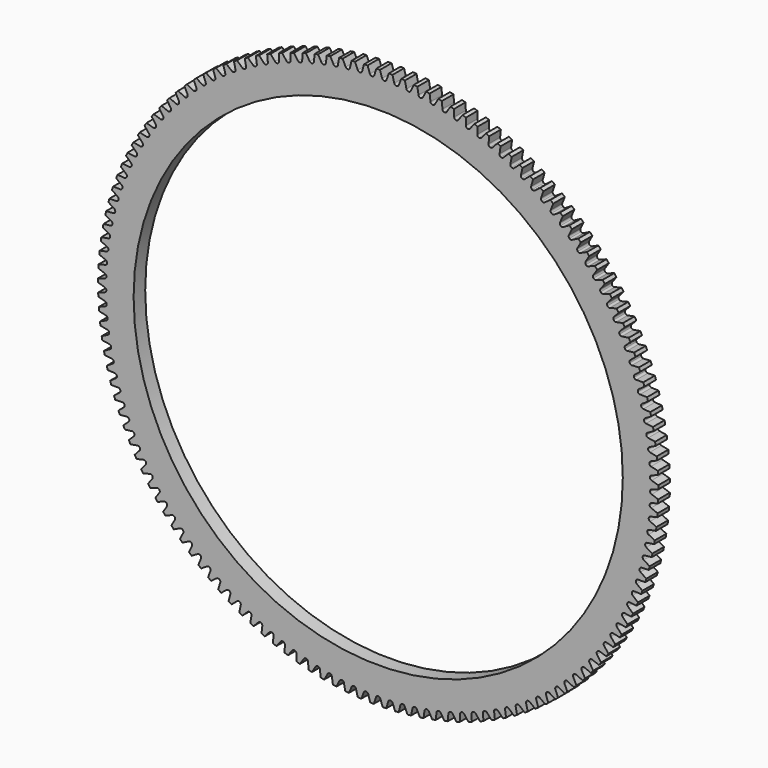
from build123d import *

# Parameters (mm, degrees)
F0_R     = 135
F1_DEPTH = 8


# Not quite as in the source:
# - ends of sketch curves that miss each other by under 0.0002 mm in the source are joined


with BuildPart() as f1:
    # F0 (on Front) → F1 (new body)
    with BuildSketch(Plane.XZ):
        with BuildLine():
            Line((2.149657, 150.904207), (1.001008, 154.59676))
            ThreePointArc((1.001008, 154.59676), (0, 154.6), (-1.0010079954, 154.5967592901))
            Line((-1.0010079954, 154.5967592901), (-2.149657, 150.904207))
            ThreePointArc((-2.149657, 150.904207), (-2.6021653574, 150.2688665421), (-3.343241, 150.025498))
            ThreePointArc((-3.343241, 150.025498), (-4.0944228128, 150.2356123099), (-4.5747845974, 150.8501647845))
            Line((-4.5747845974, 150.8501647845), (-5.886784, 154.487883))
            ThreePointArc((-5.886784, 154.487883), (-6.886942844, 154.4465280227), (-7.8868129881, 154.3986987668))
            Line((-7.8868129881, 154.3986987668), (-8.86983, 150.658644))
            ThreePointArc((-8.86983, 150.658644), (-9.2935865986, 150.003775549), (-10.0230859935, 149.7276358548))
            ThreePointArc((-10.0230859935, 149.7276358548), (-10.7828816043, 149.9040794817), (-11.2901424606, 150.4966232222))
            Line((-11.2901424606, 150.4966232222), (-12.762889, 154.072284))
            ThreePointArc((-12.762889, 154.072284), (-13.7602129304, 153.986416739), (-14.7569599887, 153.8940938824))
            Line((-14.7569599887, 153.8940938824), (-15.572393, 150.113961))
            ThreePointArc((-15.572393, 150.113961), (-15.9665572146, 149.4408662135), (-16.6830310003, 149.1325040036))
            ThreePointArc((-16.6830310003, 149.1325040036), (-17.4499321725, 149.2749258512), (-17.9830853746, 149.8442842908))
            Line((-17.9830853746, 149.8442842908), (-19.613655, 153.350789))
            ThreePointArc((-19.613655, 153.350789), (-20.6061634232, 153.2205796523), (-21.597807937, 153.0839465532))
            Line((-21.597807937, 153.0839465532), (-22.244039, 149.271242))
            ThreePointArc((-22.244039, 149.271242), (-22.6078267089, 148.5812559997), (-23.3098530061, 148.2412830456))
            ThreePointArc((-23.3098530061, 148.2412830456), (-24.0823376284, 148.3493999375), (-24.6403250099, 148.8944429949))
            Line((-24.6403250099, 148.8944429949), (-26.425479, 152.324831))
            ThreePointArc((-26.425479, 152.324831), (-27.4112015967, 152.1505373866), (-28.3957750559, 151.9698652989))
            Line((-28.3957750559, 151.9698652989), (-28.871521, 148.132158))
            ThreePointArc((-28.871521, 148.132158), (-29.2042107107, 147.4266515424), (-29.8903949713, 147.0557428405))
            ThreePointArc((-29.8903949713, 147.0557428405), (-30.6669292534, 147.1293407731), (-31.248642951, 147.6489860283))
            Line((-31.248642951, 147.6489860283), (-33.184838, 150.996446))
            ThreePointArc((-33.184838, 150.996446), (-34.1618180079, 150.7784142057), (-35.1373659455, 150.5540617666))
            Line((-35.1373659455, 150.5540617666), (-35.441681, 146.698971))
            ThreePointArc((-35.441681, 146.698971), (-35.7426132223, 145.9793450273), (-36.411593028, 145.5782371237))
            ThreePointArc((-36.411593028, 145.5782371237), (-37.1906350912, 145.6171701649), (-37.7949198522, 146.1103860945))
            Line((-37.7949198522, 146.1103860945), (-39.878311, 149.368271))
            ThreePointArc((-39.878311, 149.368271), (-40.8446086877, 149.1069345844), (-41.8091940714, 148.8393472543))
            Line((-41.8091940714, 148.8393472543), (-41.941475, 144.974527))
            ThreePointArc((-41.941475, 144.974527), (-42.2100519967, 144.2422097491), (-42.8605001177, 143.8116994298))
            ThreePointArc((-42.8605001177, 143.8116994298), (-43.6405023802, 143.8158899986), (-44.2661578786, 144.2816970855))
            Line((-44.2661578786, 144.2816970855), (-46.49261, 147.443539))
            ThreePointArc((-46.49261, 147.443539), (-47.4463065751, 147.1394168548), (-48.3980139989, 146.8291259967))
            Line((-48.3980139989, 146.8291259967), (-48.357999, 142.96225))
            ThreePointArc((-48.357999, 142.96225), (-48.5936858817, 142.218695529), (-49.2243099488, 141.7596368411))
            ThreePointArc((-49.2243099488, 141.7596368411), (-50.0037248855, 141.7290762238), (-50.649509867, 142.1665501028))
            Line((-50.649509867, 142.1665501028), (-53.014602, 145.226072))
            ThreePointArc((-53.014602, 145.226072), (-53.9538044342, 144.8797673489), (-54.8907449336, 144.5273888252))
            Line((-54.8907449336, 144.5273888252), (-54.678511, 140.666134))
            ThreePointArc((-54.678511, 140.666134), (-54.8808417827, 139.9128185145), (-55.4903900412, 139.4261231106))
            ThreePointArc((-55.4903900412, 139.4261231106), (-56.267670189, 139.3608729051), (-56.9323022426, 139.7691447946))
            Line((-56.9323022426, 139.7691447946), (-59.431339, 142.720272))
            ThreePointArc((-59.431339, 142.720272), (-60.3541820807, 142.3324724206), (-61.274495002, 141.9387060046))
            Line((-61.274495002, 141.9387060046), (-60.890465, 138.090739))
            ThreePointArc((-60.890465, 138.090739), (-61.0590363601, 137.3291573655), (-61.6462997807, 136.8157914828))
            ThreePointArc((-61.6462997807, 136.8157914828), (-62.4199014329, 136.7159810346), (-63.1020606883, 137.0942402888))
            Line((-63.1020606883, 137.0942402888), (-65.73008, 139.931114))
            ThreePointArc((-65.73008, 139.931114), (-66.6347317571, 139.5025896665), (-67.5365900447, 139.068217092))
            Line((-67.5365900447, 139.068217092), (-66.981527, 135.241177))
            ThreePointArc((-66.981527, 135.241177), (-67.116004748, 134.4728427274), (-67.6798160822, 133.9338261721))
            ThreePointArc((-67.6798160822, 133.9338261721), (-68.448203257, 133.7996526891), (-69.1465355867, 134.1471484186))
            Line((-69.1465355867, 134.1471484186), (-71.89832, 136.864136))
            ThreePointArc((-71.89832, 136.864136), (-72.7829839253, 136.3957376568), (-73.6645967253, 135.9216214931))
            Line((-73.6645967253, 135.9216214931), (-72.939602, 132.123106))
            ThreePointArc((-72.939602, 132.123106), (-73.039719853, 131.3495439601), (-73.5789597097, 130.7859464559))
            ThreePointArc((-73.5789597097, 130.7859464559), (-74.3406074994, 130.617677222), (-75.0537266479, 130.9337193899))
            Line((-75.0537266479, 130.9337193899), (-77.923812, 133.525427))
            ThreePointArc((-77.923812, 133.525427), (-78.7867323418, 133.0180845107), (-79.6463498584, 132.5051657644))
            Line((-79.6463498584, 132.5051657644), (-78.752863, 128.742718))
            ThreePointArc((-78.752863, 128.742718), (-78.8184219814, 127.9654637065), (-79.3320200625, 127.3784041055))
            ThreePointArc((-79.3320200625, 127.3784041055), (-80.0854159326, 127.1763722155), (-80.8119061154, 127.4603338601))
            Line((-80.8119061154, 127.4603338601), (-83.794594, 129.921615))
            ThreePointArc((-83.794594, 129.921615), (-84.6340575656, 129.3763359351), (-85.4699729956, 128.8256329933))
            Line((-85.4699729956, 128.8256329933), (-84.409768, 125.106722))
            ThreePointArc((-84.409768, 125.106722), (-84.4406376429, 124.3273190288), (-84.9275740807, 123.7179631234))
            ThreePointArc((-84.9275740807, 123.7179631234), (-85.6712217244, 123.4825711451), (-86.4096396772, 123.7338874287))
            Line((-86.4096396772, 123.7338874287), (-89.49901, 126.059856))
            ThreePointArc((-89.49901, 126.059856), (-90.3133495837, 125.4777226721), (-91.1239030464, 124.8903290635))
            Line((-91.1239030464, 124.8903290635), (-89.899085, 121.222339))
            ThreePointArc((-89.899085, 121.222339), (-89.8952036419, 120.4423345066), (-90.3545119051, 119.8118918681))
            ThreePointArc((-90.3545119051, 119.8118918681), (-91.0869354192, 119.5436056884), (-91.8358161037, 119.7617788486))
            Line((-91.8358161037, 119.7617788486), (-95.025734, 121.947817))
            ThreePointArc((-95.025734, 121.947817), (-95.8133327272, 121.3299850478), (-96.5969149772, 120.7070669716))
            Line((-96.5969149772, 120.7070669716), (-95.209915, 117.09728))
            ThreePointArc((-95.209915, 117.09728), (-95.1712903771, 116.3182224536), (-95.6020587486, 115.6679446817))
            ThreePointArc((-95.6020587486, 115.6679446817), (-96.3218043226, 115.3672985935), (-97.079660293, 115.5518945287))
            Line((-97.079660293, 115.5518945287), (-100.363793, 117.593661))
            ThreePointArc((-100.363793, 117.593661), (-101.1230871147, 116.9413581775), (-101.87814188, 116.284152863))
            Line((-101.87814188, 116.284152863), (-100.331715, 112.739735))
            ThreePointArc((-100.331715, 112.739735), (-100.2584245046, 111.9631717029), (-100.6597973494, 111.2943504041))
            ThreePointArc((-100.6597973494, 111.2943504041), (-101.3654352267, 110.9619395838), (-102.1307622583, 111.11259254))
            Line((-102.1307622583, 111.11259254), (-105.502588, 113.006035))
            ThreePointArc((-105.502588, 113.006035), (-106.2320709678, 112.3205550996), (-106.9571003273, 111.6303663416))
            Line((-106.9571003273, 111.6303663416), (-105.254315, 108.158356))
            ThreePointArc((-105.254315, 108.158356), (-105.1465047957, 107.3858283151), (-105.5176853011, 106.6997913183))
            ThreePointArc((-105.5176853011, 106.6997913183), (-106.2078145762, 106.3362765517), (-106.9790928527, 106.452687292))
            Line((-106.9790928527, 106.452687292), (-110.431919, 108.194045))
            ThreePointArc((-110.431919, 108.194045), (-111.1301414659, 107.4767493822), (-111.8237051815, 106.7549481733))
            Line((-111.8237051815, 106.7549481733), (-109.967943, 103.362238))
            ThreePointArc((-109.967943, 103.362238), (-109.8258253179, 102.5952799651), (-110.16607692, 101.8933889227))
            ThreePointArc((-110.16607692, 101.8933889227), (-110.8393276966, 101.4994917148), (-111.6150261855, 101.5814285874))
            Line((-111.6150261855, 101.5814285874), (-115.141996, 103.167246))
            ThreePointArc((-115.141996, 103.167246), (-115.8075727738, 102.4195591098), (-116.468294186, 101.6675781624))
            Line((-116.468294186, 101.6675781624), (-114.46324, 98.360904))
            ThreePointArc((-114.46324, 98.360904), (-114.2870972871, 97.6010385417), (-114.5957441497, 96.8846871324))
            ThreePointArc((-114.5957441497, 96.8846871324), (-115.2507797841, 96.461189931), (-116.0293581746, 96.5084905603))
            Line((-116.0293581746, 96.5084905603), (-119.623471, 97.935618))
            ThreePointArc((-119.623471, 97.935618), (-120.2550791172, 97.1590240097), (-120.8816459047, 96.378356924))
            Line((-120.8816459047, 96.378356924), (-118.73128, 93.164284))
            ThreePointArc((-118.73128, 93.164284), (-118.5214630535, 92.4130193699), (-118.7978919781, 91.6836299823))
            ThreePointArc((-118.7978919781, 91.6836299823), (-119.4334124107, 91.2313737423), (-120.2133249965, 91.2439440102))
            Line((-120.2133249965, 91.2439440102), (-123.867443, 92.509548))
            ThreePointArc((-123.867443, 92.509548), (-124.463829999, 91.7055888263), (-125.0549987572, 90.8977848235))
            Line((-125.0549987572, 90.8977848235), (-122.763591, 87.782695))
            ThreePointArc((-122.763591, 87.782695), (-122.5205160981, 87.0415226788), (-122.7641784334, 86.3005433193))
            ThreePointArc((-122.7641784334, 86.3005433193), (-123.3789207173, 85.8204254609), (-124.1586188106, 85.7982406375))
            Line((-124.1586188106, 85.7982406375), (-127.865489, 86.899809))
            ThreePointArc((-127.865489, 86.899809), (-128.4254694957, 86.0700806599), (-128.9800661266, 85.2367440837))
            Line((-128.9800661266, 85.2367440837), (-126.552166, 82.226821))
            ThreePointArc((-126.552166, 82.226821), (-126.2763149288, 81.4972130945), (-126.4867268393, 80.7461148923))
            ThreePointArc((-126.4867268393, 80.7461148923), (-127.0794716473, 80.2390882407), (-127.8574081662, 80.1821923334))
            Line((-127.8574081662, 80.1821923334), (-131.609669, 81.117538))
            ThreePointArc((-131.609669, 81.117538), (-132.1321322996, 80.2636880161), (-132.6490559667, 79.4064729801))
            Line((-132.6490559667, 79.4064729801), (-130.089483, 76.507694))
            ThreePointArc((-130.089483, 76.507694), (-129.7814040716, 75.7910982673), (-129.9581484083, 75.031372248))
            ThreePointArc((-129.9581484083, 75.031372248), (-130.5277186577, 74.4984447725), (-131.3023479981, 74.4069510095))
            Line((-131.3023479981, 74.4069510095), (-135.092551, 75.174216))
            ThreePointArc((-135.092551, 75.174216), (-135.5764588793, 74.297939391), (-136.0546831234, 73.4185480666))
            Line((-136.0546831234, 73.4185480666), (-133.368519, 70.636668))
            ThreePointArc((-133.368519, 70.636668), (-133.0288242558, 69.9345070672), (-133.1715496027, 69.1676617823))
            ThreePointArc((-133.1715496027, 69.1676617823), (-133.7168142387, 68.6098905207), (-134.4865989963, 68.4839800237))
            Line((-134.4865989963, 68.4839800237), (-138.307218, 69.081643))
            ThreePointArc((-138.307218, 69.081643), (-138.7516105774, 68.1846798203), (-139.1901860152, 67.2848580073))
            Line((-139.1901860152, 67.2848580073), (-136.382765, 64.625399))
            ThreePointArc((-136.382765, 64.625399), (-136.0121281444, 63.9390677035), (-136.120551355, 63.166625683))
            ThreePointArc((-136.120551355, 63.166625683), (-136.6404271667, 62.5851179456), (-137.4038389928, 62.4250410646))
            Line((-137.4038389928, 62.4250410646), (-141.24729, 62.851914))
            ThreePointArc((-141.24729, 62.851914), (-141.6512843299, 61.936044818), (-142.049340174, 61.0175790747))
            Line((-142.049340174, 61.0175790747), (-139.126235, 58.485822))
            ThreePointArc((-139.126235, 58.485822), (-138.7253925624, 57.8166829615), (-138.7992984203, 57.0401781838))
            ThreePointArc((-138.7992984203, 57.0401781838), (-139.2927539466, 56.4360890513), (-140.0482769559, 56.2421636668))
            Line((-140.0482769559, 56.2421636668), (-143.906928, 56.497399))
            ThreePointArc((-143.906928, 56.497399), (-144.2697222423, 55.5644422641), (-144.6264682075, 54.6291560784))
            Line((-144.6264682075, 54.6291560784), (-141.593483, 52.230127))
            ThreePointArc((-141.593483, 52.230127), (-141.1632306986, 51.5795082642), (-141.2024723009, 50.8004821159))
            ThreePointArc((-141.2024723009, 50.8004821159), (-141.6685276654, 50.1750106472), (-142.4146620087, 49.9476215959))
            Line((-142.4146620087, 49.9476215959), (-146.280852, 50.030713))
            ThreePointArc((-146.280852, 50.030713), (-146.6017260981, 49.0825213805), (-146.9164538039, 48.1322719357))
            Line((-146.9164538039, 48.1322719357), (-143.779611, 45.870734))
            ThreePointArc((-143.779611, 45.870734), (-143.3208017522, 45.2399280768), (-143.325301213, 44.4599267365))
            ThreePointArc((-143.325301213, 44.4599267365), (-143.763031174, 43.8143151756), (-144.4982949935, 43.5539137196))
            Line((-144.4982949935, 43.5539137196), (-148.364349, 43.464696))
            ThreePointArc((-148.364349, 43.464696), (-148.6426658299, 42.5031515887), (-148.914750534, 41.539825149))
            Line((-148.914750534, 41.539825149), (-145.680277, 39.420269))
            ThreePointArc((-145.680277, 39.420269), (-145.1938230494, 38.810527964), (-145.1635713185, 38.0311008051))
            ThreePointArc((-145.1635713185, 38.0311008051), (-145.5721070289, 37.3666305944), (-146.2950409965, 37.073733948))
            Line((-146.2950409965, 37.073733948), (-150.153283, 36.812384))
            ThreePointArc((-150.153283, 36.812384), (-150.3884892989, 35.8393957316), (-150.6173907722, 34.8649049473))
            Line((-150.6173907722, 34.8649049473), (-147.291709, 32.891539))
            ThreePointArc((-147.291709, 32.891539), (-146.7785755656, 32.3040730144), (-146.7136326457, 31.5267669156))
            ThreePointArc((-146.7136326457, 31.5267669156), (-147.0921627902, 30.8447577055), (-147.801331037, 30.5199473284))
            Line((-147.801331037, 30.5199473284), (-151.644101, 30.086984))
            ThreePointArc((-151.644101, 30.086984), (-151.8357303318, 29.1044840981), (-152.0209940487, 28.120764009))
            Line((-152.0209940487, 28.120764009), (-148.610706, 26.297505))
            ThreePointArc((-148.610706, 26.297505), (-148.0719128132, 25.733481014), (-147.9724081947, 24.9598400373))
            ThreePointArc((-147.9724081947, 24.9598400373), (-148.3201805466, 24.2616449664), (-149.0141759612, 23.9055657543))
            Line((-149.0141759612, 23.9055657543), (-152.833844, 23.301849))
            ThreePointArc((-152.833844, 23.301849), (-152.9815155786, 22.3117881682), (-153.122773715, 21.3207919603))
            Line((-153.122773715, 21.3207919603), (-149.634651, 19.651261))
            ThreePointArc((-149.634651, 19.651261), (-149.071267444, 19.1117974164), (-148.9373980169, 18.3433570025))
            ThreePointArc((-148.9373980169, 18.3433570025), (-149.253722927, 17.6303632434), (-149.931167105, 17.2437225143))
            Line((-149.931167105, 17.2437225143), (-153.720149, 16.470451))
            ThreePointArc((-153.720149, 16.470451), (-153.8235701646, 15.4747944035), (-153.9205423436, 14.4784890323))
            Line((-153.9205423436, 14.4784890323), (-150.36151, 12.966))
            ThreePointArc((-150.36151, 12.966), (-149.7746536674, 12.4521695459), (-149.6066857722, 11.6904549771))
            ThreePointArc((-149.6066857722, 11.6904549771), (-149.8909351733, 10.9640779286), (-150.550483004, 10.5476430159))
            Line((-150.550483004, 10.5476430159), (-154.301257, 9.606352))
            ThreePointArc((-154.301257, 9.606352), (-154.3602222943, 8.607076928), (-154.412715932, 7.6074409966))
            Line((-154.412715932, 7.6074409966), (-150.78984, 6.254997))
            ThreePointArc((-150.78984, 6.254997), (-150.1806768047, 5.7678189871), (-149.9789437229, 5.0143429845))
            ThreePointArc((-149.9789437229, 5.0143429845), (-150.2305530918, 4.2760247994), (-150.8708951802, 3.830622603))
            Line((-150.8708951802, 3.830622603), (-154.576014, 2.72318))
            ThreePointArc((-154.576014, 2.72318), (-154.5904065124, 1.7222701083), (-154.5983174023, 0.7212880019))
            Line((-154.5983174023, 0.7212880019), (-150.91879, -0.468425))
            ThreePointArc((-150.91879, -0.468425), (-150.2885295785, -0.9279830002), (-150.0534315647, -1.6717240048))
            ThreePointArc((-150.0534315647, -1.6717240048), (-150.2719016623, -2.420518241), (-150.8917670127, -2.8940039637))
            Line((-150.8917670127, -2.8940039637), (-154.543875, -4.165398))
            ThreePointArc((-154.543875, -4.165398), (-154.5136657576, -5.1659552992), (-154.4769781992, -6.1662960079))
            Line((-154.4769781992, -6.1662960079), (-150.748106, -7.190917))
            ThreePointArc((-150.748106, -7.190917), (-150.0979991028, -7.6219421325), (-149.8300030546, -8.3544720018))
            ThreePointArc((-149.8300030546, -8.3544720018), (-150.0149002819, -9.112255131), (-150.6130580665, -9.6128838333))
            Line((-150.6130580665, -9.6128838333), (-154.204904, -11.045706))
            ThreePointArc((-154.204904, -11.045706), (-154.1301524147, -12.0439244689), (-154.0489392296, -13.0416380194))
            Line((-154.0489392296, -13.0416380194), (-150.278125, -13.899132))
            ThreePointArc((-150.278125, -13.899132), (-149.6094628198, -14.3007697005), (-149.309100919, -15.0206339937))
            ThreePointArc((-149.309100919, -15.0206339937), (-149.4600572607, -15.7859012926), (-150.0353200934, -16.3126787932))
            Line((-150.0353200934, -16.3126787932), (-153.559772, -17.904084))
            ThreePointArc((-153.559772, -17.904084), (-153.4406279523, -18.8979812041), (-153.315050453, -19.8910860588))
            Line((-153.315050453, -19.8910860588), (-149.509781, -20.579751))
            ThreePointArc((-149.509781, -20.579751), (-148.8238913542, -20.9512038922), (-148.491760025, -21.6569731262))
            ThreePointArc((-148.491760025, -21.6569731262), (-148.6084751738, -22.4282055726), (-149.1597007065, -22.9800865796))
            Line((-149.1597007065, -22.9800865796), (-152.609763, -24.726915))
            ThreePointArc((-152.609763, -24.726915), (-152.4464612925, -25.7145180665), (-152.2767687333, -26.7010431286))
            Line((-152.2767687333, -26.7010431286), (-148.444599, -27.219512))
            ThreePointArc((-148.444599, -27.219512), (-147.7428423662, -27.5600409242), (-147.3796010638, -28.2503150108))
            ThreePointArc((-147.3796010638, -28.2503150108), (-147.4618457463, -29.0259807861), (-147.9879389954, -29.6018690081))
            Line((-147.9879389954, -29.6018690081), (-151.35676, -31.500653))
            ThreePointArc((-151.35676, -31.500653), (-151.149626225, -32.4800014169), (-150.9361554825, -33.457988107))
            Line((-150.9361554825, -33.457988107), (-147.084694, -33.80523))
            ThreePointArc((-147.084694, -33.80523), (-146.3684648034, -34.1141607975), (-145.9748345203, -34.7875681118))
            ThreePointArc((-145.9748345203, -34.7875681118), (-146.0224435401, -35.5661277291), (-146.5223609573, -36.1648800685))
            Line((-146.5223609573, -36.1648800685), (-149.803253, -38.211849))
            ThreePointArc((-149.803253, -38.211849), (-149.5526977476, -39.1809978996), (-149.2958727193, -40.1485041934))
            Line((-149.2958727193, -40.1485041934), (-145.432765, -40.323832))
            ThreePointArc((-145.432765, -40.323832), (-144.7034855151, -40.6005495393), (-144.2802482629, -41.2557530689))
            ThreePointArc((-144.2802482629, -41.2557530689), (-144.2931272152, -42.0356610236), (-144.7658758918, -42.6560891574))
            Line((-144.7658758918, -42.6560891574), (-147.952325, -44.847179))
            ThreePointArc((-147.952325, -44.847179), (-147.6588460822, -45.8042047599), (-147.3591765454, -46.7593101731))
            Line((-147.3591765454, -46.7593101731), (-143.492094, -46.762374))
            ThreePointArc((-143.492094, -46.762374), (-142.7512115618, -47.0063303619), (-142.2992069496, -47.6420292946))
            ThreePointArc((-142.2992069496, -47.6420292946), (-142.2773308332, -48.4217366018), (-142.721971863, -49.0626081814))
            Line((-142.721971863, -49.0626081814), (-145.807651, -51.393469))
            ThreePointArc((-145.807651, -51.393469), (-145.4718315365, -52.3364713123), (-145.1299125624, -53.2772792064))
            Line((-145.1299125624, -53.2772792064), (-141.266532, -53.108074))
            ThreePointArc((-141.266532, -53.108074), (-140.5155174859, -53.3187836797), (-140.0356429661, -53.9337159878))
            ThreePointArc((-140.0356429661, -53.9337159878), (-139.9790552513, -54.7116748267), (-140.3947064242, -55.3717174876))
            Line((-140.3947064242, -55.3717174876), (-143.37349, -57.837723))
            ThreePointArc((-143.37349, -57.837723), (-142.9959959871, -58.7648290361), (-142.6125065494, -59.6894712299))
            Line((-142.6125065494, -59.6894712299), (-138.760499, -59.348333))
            ThreePointArc((-138.760499, -59.348333), (-138.0008432724, -59.5253774597), (-137.4940518053, -60.11832292))
            ThreePointArc((-137.4940518053, -60.11832292), (-137.4028652002, -60.8929885552), (-137.7887001221, -61.5708918652))
            Line((-137.7887001221, -61.5708918652), (-140.654675, -64.167145))
            ThreePointArc((-140.654675, -64.167145), (-140.2362552913, -65.0765142112), (-139.8119566309, -65.9831552977))
            Line((-139.8119566309, -65.9831552977), (-135.97897, -65.470761))
            ThreePointArc((-135.97897, -65.470761), (-135.2121813349, -65.6137897984), (-134.6794791214, -66.1835710564))
            ThreePointArc((-134.6794791214, -66.1835710564), (-134.5538736811, -66.9534054012), (-134.9091276137, -67.64782339))
            Line((-134.9091276137, -67.64782339), (-137.656602, -70.369168))
            ThreePointArc((-137.656602, -70.369168), (-137.1980886021, -71.2589958105), (-136.7338229876, -72.1458359935))
            Line((-136.7338229876, -72.1458359935), (-132.927467, -71.463202))
            ThreePointArc((-132.927467, -71.463202), (-132.1550678523, -71.5719315693), (-131.5975122152, -72.1174165924))
            ThreePointArc((-131.5975122152, -72.1174165924), (-131.4377377772, -72.8808917225), (-131.7617049129, -73.5904460804))
            Line((-131.7617049129, -73.5904460804), (-134.385225, -76.431481))
            ThreePointArc((-134.385225, -76.431481), (-133.8875275161, -77.2999998423), (-133.3842169176, -78.1652779517))
            Line((-133.3842169176, -78.1652779517), (-129.612048, -77.313761))
            ThreePointArc((-129.612048, -77.313761), (-128.8355726032, -77.3879738524), (-128.254271184, -77.9080801062))
            ThreePointArc((-128.254271184, -77.9080801062), (-128.0606454146, -78.6636795518), (-128.3526822462, -79.3869607922))
            Line((-128.3526822462, -79.3869607922), (-130.847038, -82.342046))
            ThreePointArc((-130.847038, -82.342046), (-130.3111451491, -83.1875318178), (-129.7697888666, -84.0295299136))
            Line((-129.7697888666, -84.0295299136), (-126.039297, -83.01082))
            ThreePointArc((-126.039297, -83.01082), (-125.2602866122, -83.0503705363), (-124.656393496, -83.5440653166))
            ThreePointArc((-124.656393496, -83.5440653166), (-124.4292993343, -84.2902890867), (-124.6888270562, -85.0258619567))
            Line((-124.6888270562, -85.0258619567), (-127.049067, -88.089128))
            ThreePointArc((-127.049067, -88.089128), (-126.4760422903, -88.9099022977), (-125.8977149498, -89.7269489642))
            Line((-125.8977149498, -89.7269489642), (-122.216307, -88.543069))
            ThreePointArc((-122.216307, -88.543069), (-121.4363076018, -88.5478763835), (-120.8110207229, -89.0141798052))
            ThreePointArc((-120.8110207229, -89.0141798052), (-120.5509113922, -89.7495470908), (-120.7774134377, -90.4959506928))
            Line((-120.7774134377, -90.4959506928), (-122.998852, -93.661318))
            ThreePointArc((-122.998852, -93.661318), (-122.3898327712, -94.455750668), (-121.7756827074, -95.2462235533))
            Line((-121.7756827074, -95.2462235533), (-118.150667, -93.899523))
            ThreePointArc((-118.150667, -93.899523), (-117.3712281837, -93.8695807067), (-116.7257904108, -94.307566317))
            ThreePointArc((-116.7257904108, -94.307566317), (-116.4331795848, -95.0306159799), (-116.6262070849, -95.7863689459))
            Line((-116.6262070849, -95.7863689459), (-118.704433, -99.047551))
            ThreePointArc((-118.704433, -99.047551), (-118.0606297325, -99.814065678), (-117.4118763511, -100.5763953008))
            Line((-117.4118763511, -100.5763953008), (-113.850451, -99.069549))
            ThreePointArc((-113.850451, -99.069549), (-113.0731193685, -99.0049145049), (-112.4088109482, -99.4137129562))
            ThreePointArc((-112.4088109482, -99.4137129562), (-112.0842818977, -100.1230098896), (-112.2434512491, -100.8866108564))
            Line((-112.2434512491, -100.8866108564), (-114.174338, -104.237135))
            ThreePointArc((-114.174338, -104.237135), (-113.4970280329, -104.9742093454), (-112.8149592919, -105.7068822735))
            Line((-112.8149592919, -105.7068822735), (-109.324194, -104.042881))
            ThreePointArc((-109.324194, -104.042881), (-108.5505135689, -103.9436835429), (-107.868654343, -104.3224833172))
            ThreePointArc((-107.868654343, -104.3224833172), (-107.5128504772, -105.0166195171), (-107.6378459243, -105.7865530393))
            Line((-107.6378459243, -105.7865530393), (-109.417561, -109.219766))
            ThreePointArc((-109.417561, -109.219766), (-108.7080884367, -109.9259364684), (-107.9940582778, -110.6274982845))
            Line((-107.9940582778, -110.6274982845), (-104.580885, -108.809646))
            ThreePointArc((-104.580885, -108.809646), (-103.8123915438, -108.6760816476), (-103.1143347378, -109.0241307349))
            ThreePointArc((-103.1143347378, -109.0241307349), (-102.7279626122, -109.7017282096), (-102.8185357114, -110.4764656706))
            Line((-102.8185357114, -110.4764656706), (-104.443545, -113.985551))
            ThreePointArc((-104.443545, -113.985551), (-103.7033193289, -114.6594154885), (-102.9587458656, -115.3284728494))
            Line((-102.9587458656, -115.3284728494), (-99.62994, -113.36038))
            ThreePointArc((-99.62994, -113.36038), (-98.8681594996, -113.1927134146), (-98.1552909736, -113.5093209708))
            ThreePointArc((-98.1552909736, -113.5093209708), (-97.7391176603, -114.1690339884), (-97.7950883016, -114.9470368763))
            Line((-97.7950883016, -114.9470368763), (-99.262166, -118.525028))
            ThreePointArc((-99.262166, -118.525028), (-98.4926566867, -119.1652490401), (-97.7190178988, -119.8004738759))
            Line((-97.7190178988, -119.8004738759), (-94.481189, -117.686047))
            ThreePointArc((-94.481189, -117.686047), (-93.727633832, -117.484612375), (-93.0013693527, -117.7691494268))
            ThreePointArc((-93.0013693527, -117.7691494268), (-92.5562198778, -118.4096676863), (-92.5774777458, -119.1893920912))
            Line((-92.5774777458, -119.1893920912), (-93.883711, -122.829185))
            ThreePointArc((-93.883711, -122.829185), (-93.0864458965, -123.4344910889), (-92.2852780189, -124.0346220254))
            Line((-92.2852780189, -124.0346220254), (-89.144854, -121.778059))
            ThreePointArc((-89.144854, -121.778059), (-88.4010202208, -121.5432551863), (-87.6628012191, -121.7951572906))
            ThreePointArc((-87.6628012191, -121.7951572906), (-87.1895610542, -122.4152104816), (-87.1760639994, -123.1951080002))
            Line((-87.1760639994, -123.1951080002), (-88.318859, -126.889476))
            ThreePointArc((-88.318859, -126.889476), (-87.4954206166, -127.4586653434), (-86.6683140465, -128.0225110687))
            Line((-86.6683140465, -128.0225110687), (-83.631531, -125.628292))
            ThreePointArc((-83.631531, -125.628292), (-82.8988947265, -125.360586594), (-82.1501870654, -125.5793530953))
            ThreePointArc((-82.1501870654, -125.5793530953), (-81.6497956461, -126.1777093871), (-81.6015697212, -126.9562310728))
            Line((-81.6015697212, -126.9562310728), (-82.578658, -130.697839))
            ThreePointArc((-82.578658, -130.697839), (-81.7306814147, -131.2297821209), (-80.8792781539, -131.7562232507))
            Line((-80.8792781539, -131.7562232507), (-77.952165, -129.229102))
            ThreePointArc((-77.952165, -129.229102), (-77.2321816308, -128.9290254641), (-76.4744718488, -129.1142217573))
            ThreePointArc((-76.4744718488, -129.1142217573), (-75.9479216868, -129.6896930632), (-75.8650629382, -130.4652940132))
            Line((-75.8650629382, -130.4652940132), (-76.674505, -134.246714))
            ThreePointArc((-76.674505, -134.246714), (-75.8036736669, -134.7403542321), (-74.929664253, -135.2283454566))
            Line((-74.929664253, -135.2283454566), (-72.118032, -132.573339))
            ThreePointArc((-72.118032, -132.573339), (-71.4121306161, -132.2414874968), (-70.6469230098, -132.3927470174))
            ThreePointArc((-70.6469230098, -132.3927470174), (-70.095260756, -132.9441906708), (-69.9779338374, -133.7153300273))
            Line((-69.9779338374, -133.7153300273), (-70.618121, -137.529055))
            ThreePointArc((-70.618121, -137.529055), (-69.7261642125, -137.9834121343), (-68.8312842142, -138.4319844307))
            Line((-68.8312842142, -138.4319844307), (-66.140715, -135.654364))
            ThreePointArc((-66.140715, -135.654364), (-65.450297672, -135.2913959629), (-64.6791116487, -135.4084173047))
            ThreePointArc((-64.6791116487, -135.4084173047), (-64.1034319004, -135.9347394879), (-63.9518692416, -136.6998869704))
            Line((-63.9518692416, -136.6998869704), (-64.421532, -140.538344))
            ThreePointArc((-64.421532, -140.538344), (-63.5102204457, -140.952516469), (-62.5962461928, -141.3607794354))
            Line((-62.5962461928, -141.3607794354), (-60.032082, -138.46606))
            ThreePointArc((-60.032082, -138.46606), (-59.358519165, -138.072696675), (-58.5828859798, -138.1552479552))
            ThreePointArc((-58.5828859798, -138.1552479552), (-57.9843312746, -138.6554025274), (-57.7988341081, -139.4130389916))
            Line((-57.7988341081, -139.4130389916), (-58.09704, -143.268607))
            ThreePointArc((-58.09704, -143.268607), (-57.1681830982, -143.6417726194), (-56.2369292555, -144.0089156542))
            Line((-56.2369292555, -144.0089156542), (-53.804261, -141.002845))
            ThreePointArc((-53.804261, -141.002845), (-53.1488899766, -140.5798668841), (-52.3703492125, -140.627784534))
            ThreePointArc((-52.3703492125, -140.627784534), (-51.7501083368, -141.1007779978), (-51.5310453474, -141.8493989887))
            Line((-51.5310453474, -141.8493989887), (-51.657201, -145.714424))
            ThreePointArc((-51.657201, -145.714424), (-50.7126427914, -146.0458416427), (-49.765958274, -146.3711358058))
            Line((-49.765958274, -146.3711358058), (-47.469616, -143.259681))
            ThreePointArc((-47.469616, -143.259681), (-46.8337383145, -142.8079282052), (-46.0538361891, -142.8211165447))
            ThreePointArc((-46.0538361891, -142.8211165447), (-45.4131402778, -143.266011245), (-45.1609459861, -144.0041309998))
            Line((-45.1609459861, -144.0041309998), (-45.114802, -147.870939))
            ThreePointArc((-45.114802, -147.870939), (-44.1564176803, -148.1599499786), (-43.1961821174, -148.4427494035))
            Line((-43.1961821174, -148.4427494035), (-41.040725, -145.232088))
            ThreePointArc((-41.040725, -145.232088), (-40.4256021371, -144.7524581026), (-39.6458870319, -144.7308911071))
            ThreePointArc((-39.6458870319, -144.7308911071), (-38.9860092929, -145.1468033438), (-38.701184261, -145.8729550148))
            Line((-38.701184261, -145.8729550148), (-38.482832, -149.733869))
            ThreePointArc((-38.482832, -149.733869), (-37.5125244546, -149.9799003502), (-36.5406441475, -150.2196436066))
            Line((-36.5406441475, -150.2196436066), (-34.530352, -146.916151))
            ThreePointArc((-34.530352, -146.916151), (-33.9372059425, -146.4095946378), (-33.1592250588, -146.3533152351))
            ThreePointArc((-33.1592250588, -146.3533152351), (-32.4814742537, -146.7394187319), (-32.1645842536, -147.4521620257))
            Line((-32.1645842536, -147.4521620257), (-31.774457, -151.299517))
            ThreePointArc((-31.774457, -151.299517), (-30.7941530778, -151.5020796432), (-29.8125581226, -151.6982906238))
            Line((-29.8125581226, -151.6982906238), (-27.951422, -148.308525))
            ThreePointArc((-27.951422, -148.308525), (-27.3814294351, -147.7760490995), (-26.6067279553, -147.68516878))
            ThreePointArc((-26.6067279553, -147.68516878), (-25.9124508227, -148.0406978896), (-25.5641253356, -148.7386170492))
            Line((-25.5641253356, -148.7386170492), (-25.002997, -152.564773))
            ThreePointArc((-25.002997, -152.564773), (-24.0146429943, -152.7234655246), (-23.0252821097, -152.8757547284))
            Line((-23.0252821097, -152.8757547284), (-21.316996, -149.406447))
            ThreePointArc((-21.316996, -149.406447), (-20.7712903422, -148.8491077613), (-20.0014060871, -148.7238075539))
            ThreePointArc((-20.0014060871, -148.7238075539), (-19.2919803314, -149.0480557975), (-18.9129101064, -149.7297650205))
            Line((-18.9129101064, -149.7297650205), (-18.181897, -153.527126))
            ThreePointArc((-18.181897, -153.527126), (-17.1874543337, -153.6416330736), (-16.1922910261, -153.7496982479))
            Line((-16.1922910261, -153.7496982479), (-14.640248, -150.207736))
            ThreePointArc((-14.640248, -150.207736), (-14.1199112027, -149.6266407922), (-13.3563730827, -149.4671687388))
            ThreePointArc((-13.3563730827, -149.4671687388), (-12.6332075513, -149.7594919945), (-12.224145775, -150.4236379462))
            Line((-12.224145775, -150.4236379462), (-11.324697, -154.184666))
            ThreePointArc((-11.324697, -154.184666), (-10.3261409543, -154.25475945), (-9.3271519957, -154.3183859287))
            Line((-9.3271519957, -154.3183859287), (-7.934433, -150.710801))
            ThreePointArc((-7.934433, -150.710801), (-7.4404988381, -150.1071035081), (-6.6848230232, -149.9137763471))
            ThreePointArc((-6.6848230232, -149.9137763471), (-5.9493528319, -150.1735946072), (-5.5111111607, -150.8188590461))
            Line((-5.5111111607, -150.8188590461), (-4.445014, -154.536086))
            ThreePointArc((-4.445014, -154.536086), (-3.4443267043, -154.5616272351), (-2.4434950117, -154.5806887426))
            Line((-2.4434950117, -154.5806887426), (-1.212865, -150.914644))
            ThreePointArc((-1.212865, -150.914644), (-0.7463141639, -150.2895421151), (-5.9e-09, -150.0627442651))
            ThreePointArc((-5.9e-09, -150.0627442651), (0.7463141639, -150.2895421151), (1.2128650742, -150.9146439751))
            Line((1.2128650742, -150.9146439751), (2.443495, -154.580688))
            ThreePointArc((2.443495, -154.580688), (3.4443267043, -154.5616272351), (4.4450139976, -154.536085917))
            Line((4.4450139976, -154.536085917), (5.511112, -150.818859))
            ThreePointArc((5.511112, -150.818859), (5.9493534361, -150.1735949124), (6.6848230059, -149.9137762651))
            ThreePointArc((6.6848230059, -149.9137762651), (7.4404992657, -150.1071031429), (7.9344333149, -150.7108008784))
            Line((7.9344333149, -150.7108008784), (9.327152, -154.318386))
            ThreePointArc((9.327152, -154.318386), (10.3261414519, -154.2547594167), (11.3246979966, -154.1846659538))
            Line((11.3246979966, -154.1846659538), (12.224146, -150.423638))
            ThreePointArc((12.224146, -150.423638), (12.6332079324, -149.7594916725), (13.3563740232, -149.4671683471))
            ThreePointArc((13.3563740232, -149.4671683471), (14.1199120288, -149.6266406919), (14.6402484123, -150.2077358193))
            Line((14.6402484123, -150.2077358193), (16.192291, -153.749698))
            ThreePointArc((16.192291, -153.749698), (17.1874543337, -153.6416330736), (18.1818970775, -153.5271266541))
            Line((18.1818970775, -153.5271266541), (18.912911, -149.729765))
            ThreePointArc((18.912911, -149.729765), (19.2919809664, -149.0480561348), (20.001406095, -148.7238078493))
            ThreePointArc((20.001406095, -148.7238078493), (20.7712905382, -148.8491078631), (21.3169965937, -149.4064472001))
            Line((21.3169965937, -149.4064472001), (23.025282, -152.875754))
            ThreePointArc((23.025282, -152.875754), (24.0146434818, -152.723465448), (25.0029980682, -152.5647734164))
            Line((25.0029980682, -152.5647734164), (25.564125, -148.738617))
            ThreePointArc((25.564125, -148.738617), (25.9124508227, -148.0406978896), (26.6067279337, -147.685168578))
            ThreePointArc((26.6067279337, -147.685168578), (27.3814297722, -147.7760487922), (27.9514218798, -148.308525066))
            Line((27.9514218798, -148.308525066), (29.812558, -151.69829))
            ThreePointArc((29.812558, -151.69829), (30.7941535573, -151.5020795457), (31.774457983, -151.2995169189))
            Line((31.774457983, -151.2995169189), (32.164585, -147.452162))
            ThreePointArc((32.164585, -147.452162), (32.4814749249, -146.7394190951), (33.1592249949, -146.3533149751))
            ThreePointArc((33.1592249949, -146.3533149751), (33.9372059425, -146.4095946378), (34.5303520576, -146.916150965))
            Line((34.5303520576, -146.916150965), (36.540645, -150.219643))
            ThreePointArc((36.540645, -150.219643), (37.5125249259, -149.9799002323), (38.482832093, -149.7338693619))
            Line((38.482832093, -149.7338693619), (38.701184, -145.872955))
            ThreePointArc((38.701184, -145.872955), (38.9860092929, -145.1468033438), (39.6458870588, -144.7308912351))
            ThreePointArc((39.6458870588, -144.7308912351), (40.4256026861, -144.7524579405), (41.0407256683, -145.2320882227))
            Line((41.0407256683, -145.2320882227), (43.196183, -148.442749))
            ThreePointArc((43.196183, -148.442749), (44.1564181403, -148.1599498414), (45.1148020375, -147.870939123))
            Line((45.1148020375, -147.870939123), (45.160947, -144.004131))
            ThreePointArc((45.160947, -144.004131), (45.4131409891, -143.2660116275), (46.0538361135, -142.8211163808))
            ThreePointArc((46.0538361135, -142.8211163808), (46.8337385981, -142.807928293), (47.4696167475, -143.2596811863))
            Line((47.4696167475, -143.2596811863), (49.765959, -146.371135))
            ThreePointArc((49.765959, -146.371135), (50.7126436837, -146.0458413328), (51.6572021295, -145.7144243654))
            Line((51.6572021295, -145.7144243654), (51.531046, -141.849399))
            ThreePointArc((51.531046, -141.849399), (51.7501083276, -141.1007780112), (52.3703488793, -140.6277836523))
            ThreePointArc((52.3703488793, -140.6277836523), (53.1488899766, -140.5798668841), (53.804261252, -141.002844796))
            Line((53.804261252, -141.002844796), (56.236929, -144.008915))
            ThreePointArc((56.236929, -144.008915), (57.1681830982, -143.6417726194), (58.0970402328, -143.268607574))
            Line((58.0970402328, -143.268607574), (57.798835, -139.413039))
            ThreePointArc((57.798835, -139.413039), (57.9843320288, -138.6554029216), (58.5828862125, -138.155248534))
            ThreePointArc((58.5828862125, -138.155248534), (59.358519165, -138.072696675), (60.0320819289, -138.466060063))
            Line((60.0320819289, -138.466060063), (62.596246, -141.360779))
            ThreePointArc((62.596246, -141.360779), (63.5102204457, -140.952516469), (64.4215321085, -140.5383442367))
            Line((64.4215321085, -140.5383442367), (63.95187, -136.699887))
            ThreePointArc((63.95187, -136.699887), (64.1034318706, -135.9347395408), (64.6791119798, -135.4084179552))
            ThreePointArc((64.6791119798, -135.4084179552), (65.4502978888, -135.2913958311), (66.1407155073, -135.6543635086))
            Line((66.1407155073, -135.6543635086), (68.831284, -138.431984))
            ThreePointArc((68.831284, -138.431984), (69.7261646095, -137.9834119336), (70.6181218168, -137.5290546432))
            Line((70.6181218168, -137.5290546432), (69.977934, -133.71533))
            ThreePointArc((69.977934, -133.71533), (70.095260756, -132.9441906708), (70.6469228521, -132.3927467073))
            ThreePointArc((70.6469228521, -132.3927467073), (71.4121306161, -132.2414874968), (72.1180319143, -132.5733390908))
            Line((72.1180319143, -132.5733390908), (74.929664, -135.228345))
            ThreePointArc((74.929664, -135.228345), (75.8036736669, -134.7403542321), (76.6745051014, -134.2467141775))
            Line((76.6745051014, -134.2467141775), (75.865064, -130.465294))
            ThreePointArc((75.865064, -130.465294), (75.9479225077, -129.6896934605), (76.4744720098, -129.1142220174))
            ThreePointArc((76.4744720098, -129.1142220174), (77.2321818304, -128.9290254019), (77.9521651606, -129.229101814))
            Line((77.9521651606, -129.229101814), (80.879278, -131.756223))
            ThreePointArc((80.879278, -131.756223), (81.7306814147, -131.2297821209), (82.5786582136, -130.6978393381))
            Line((82.5786582136, -130.6978393381), (81.60157, -126.956231))
            ThreePointArc((81.60157, -126.956231), (81.6497958032, -126.1777089928), (82.1501878488, -125.5793527573))
            ThreePointArc((82.1501878488, -125.5793527573), (82.8988951385, -125.3605866076), (83.6315308093, -125.6282922418))
            Line((83.6315308093, -125.6282922418), (86.668314, -128.022511))
            ThreePointArc((86.668314, -128.022511), (87.495420955, -127.4586651111), (88.3188597205, -126.8894755985))
            Line((88.3188597205, -126.8894755985), (87.176064, -123.195108))
            ThreePointArc((87.176064, -123.195108), (87.1895611895, -122.4152100922), (87.6628017451, -121.7951566287))
            ThreePointArc((87.6628017451, -121.7951566287), (88.401021026, -121.543255177), (89.14485519, -121.7780587356))
            Line((89.14485519, -121.7780587356), (92.285278, -124.034622))
            ThreePointArc((92.285278, -124.034622), (93.0864462136, -123.4344908497), (93.8837118691, -122.8291848287))
            Line((93.8837118691, -122.8291848287), (92.577478, -119.189392))
            ThreePointArc((92.577478, -119.189392), (92.5562208119, -118.409667907), (93.0013692191, -117.7691492906))
            ThreePointArc((93.0013692191, -117.7691492906), (93.727633832, -117.484612375), (94.4811891442, -117.6860467792))
            Line((94.4811891442, -117.6860467792), (97.719018, -119.800474))
            ThreePointArc((97.719018, -119.800474), (98.4926566867, -119.1652490401), (99.2621662878, -118.5250283436))
            Line((99.2621662878, -118.5250283436), (97.795089, -114.947037))
            ThreePointArc((97.795089, -114.947037), (97.7391176142, -114.1690341724), (98.1552913527, -113.5093214268))
            ThreePointArc((98.1552913527, -113.5093214268), (98.8681594996, -113.1927134146), (99.6299402776, -113.3603795304))
            Line((99.6299402776, -113.3603795304), (102.958746, -115.328473))
            ThreePointArc((102.958746, -115.328473), (103.7033193289, -114.6594154885), (104.4435451553, -113.9855511694))
            Line((104.4435451553, -113.9855511694), (102.818536, -110.476466))
            ThreePointArc((102.818536, -110.476466), (102.7279625703, -109.7017284155), (103.1143349736, -109.0241309708))
            ThreePointArc((103.1143349736, -109.0241309708), (103.8123915438, -108.6760816476), (104.5808848484, -108.8096462846))
            Line((104.5808848484, -108.8096462846), (107.994059, -110.627498))
            ThreePointArc((107.994059, -110.627498), (108.7080886911, -109.9259362168), (109.4175611367, -109.2197661364))
            Line((109.4175611367, -109.2197661364), (107.637846, -105.786553))
            ThreePointArc((107.637846, -105.786553), (107.5128505325, -105.0166191659), (107.8686547378, -104.3224827349))
            ThreePointArc((107.8686547378, -104.3224827349), (108.5505145689, -103.9436835429), (109.3241947595, -104.0428815044))
            Line((109.3241947595, -104.0428815044), (112.814959, -105.706882))
            ThreePointArc((112.814959, -105.706882), (113.4970282618, -104.9742090979), (114.1743390022, -104.237135002))
            Line((114.1743390022, -104.237135002), (112.243451, -100.886611))
            ThreePointArc((112.243451, -100.886611), (112.0842818977, -100.1230098896), (112.4088108445, -99.4137128562))
            ThreePointArc((112.4088108445, -99.4137128562), (113.0731196066, -99.0049146868), (113.8504509659, -99.0695490807))
            Line((113.8504509659, -99.0695490807), (117.411876, -100.576395))
            ThreePointArc((117.411876, -100.576395), (118.0606299393, -99.8140654334), (118.7044339743, -99.0475509785))
            Line((118.7044339743, -99.0475509785), (116.626208, -95.786369))
            ThreePointArc((116.626208, -95.786369), (116.4331805848, -95.0306159799), (116.7257909482, -94.3075659562))
            ThreePointArc((116.7257909482, -94.3075659562), (117.371228928, -93.8695804936), (118.1506678103, -93.8995235107))
            Line((118.1506678103, -93.8995235107), (121.775683, -95.246223))
            ThreePointArc((121.775683, -95.246223), (122.3898329594, -94.4557504241), (122.9988517869, -93.6613178377))
            Line((122.9988517869, -93.6613178377), (120.777414, -90.495951))
            ThreePointArc((120.777414, -90.495951), (120.5509113926, -89.7495470725), (120.8110217841, -89.0141798334))
            ThreePointArc((120.8110217841, -89.0141798334), (121.4363081505, -88.5478765348), (122.216307339, -88.543067946))
            Line((122.216307339, -88.543067946), (125.897715, -89.726949))
            ThreePointArc((125.897715, -89.726949), (126.4760422903, -88.9099022977), (127.0490672728, -88.0891281891))
            Line((127.0490672728, -88.0891281891), (124.688827, -85.025862))
            ThreePointArc((124.688827, -85.025862), (124.4293003276, -84.2902887816), (124.6563937229, -83.5440648052))
            ThreePointArc((124.6563937229, -83.5440648052), (125.2602873133, -83.0503702659), (126.0392979321, -83.0108202487))
            Line((126.0392979321, -83.0108202487), (129.769789, -84.02953))
            ThreePointArc((129.769789, -84.02953), (130.3111452924, -83.1875315933), (130.847038577, -82.3420457338))
            Line((130.847038577, -82.3420457338), (128.352683, -79.386961))
            ThreePointArc((128.352683, -79.386961), (128.0606454181, -78.6636796052), (128.2542717855, -77.9080798631))
            ThreePointArc((128.2542717855, -77.9080798631), (128.835573279, -77.3879735566), (129.6120490718, -77.3137606817))
            Line((129.6120490718, -77.3137606817), (133.384217, -78.165278))
            ThreePointArc((133.384217, -78.165278), (133.8875275161, -77.2999998423), (134.3852250389, -76.4314810221))
            Line((134.3852250389, -76.4314810221), (131.761706, -73.590446))
            ThreePointArc((131.761706, -73.590446), (131.4377388049, -72.880891971), (131.597513184, -72.1174171062))
            ThreePointArc((131.597513184, -72.1174171062), (132.1550682039, -71.5719318883), (132.9274668993, -71.4632025617))
            Line((132.9274668993, -71.4632025617), (136.733823, -72.145836))
            ThreePointArc((136.733823, -72.145836), (137.1980886021, -71.2589958105), (137.6566023479, -70.3691681778))
            Line((137.6566023479, -70.3691681778), (134.909128, -67.647823))
            ThreePointArc((134.909128, -67.647823), (134.5538736811, -66.9534054012), (134.6794790027, -66.1835710014))
            ThreePointArc((134.6794790027, -66.1835710014), (135.2121813349, -65.6137897984), (135.9789700643, -65.4707605193))
            Line((135.9789700643, -65.4707605193), (139.811957, -65.983155))
            ThreePointArc((139.811957, -65.983155), (140.2362553811, -65.0765140177), (140.6546747152, -64.1671448701))
            Line((140.6546747152, -64.1671448701), (137.788701, -61.570892))
            ThreePointArc((137.788701, -61.570892), (137.4028652739, -60.8929889183), (137.4940525033, -60.1183232335))
            ThreePointArc((137.4940525033, -60.1183232335), (138.0008436844, -59.5253778171), (138.7604990703, -59.3483322064))
            Line((138.7604990703, -59.3483322064), (142.612507, -59.689471))
            ThreePointArc((142.612507, -59.689471), (142.9959961316, -58.7648286846), (143.37349063, -57.8377228508))
            Line((143.37349063, -57.8377228508), (140.394707, -55.371718))
            ThreePointArc((140.394707, -55.371718), (139.9790562974, -54.7116750111), (140.0356436608, -53.9337162716))
            ThreePointArc((140.0356436608, -53.9337162716), (140.5155183453, -53.318783774), (141.2665329936, -53.1080741464))
            Line((141.2665329936, -53.1080741464), (145.129913, -53.277279))
            ThreePointArc((145.129913, -53.277279), (145.4718316511, -52.3364709938), (145.8076518853, -51.3934689596))
            Line((145.8076518853, -51.3934689596), (142.721972, -49.062608))
            ThreePointArc((142.721972, -49.062608), (142.2773307849, -48.4217364396), (142.2992069661, -47.6420289878))
            ThreePointArc((142.2992069661, -47.6420289878), (142.7512116811, -47.006330274), (143.4920940003, -46.7623743928))
            Line((143.4920940003, -46.7623743928), (147.359177, -46.75931))
            ThreePointArc((147.359177, -46.75931), (147.658846127, -45.8042046154), (147.9523251945, -44.847179059))
            Line((147.9523251945, -44.847179059), (144.765876, -42.656089))
            ThreePointArc((144.765876, -42.656089), (144.2931272152, -42.0356610236), (144.2802480374, -41.2557530116))
            ThreePointArc((144.2802480374, -41.2557530116), (144.7034859035, -40.6005492252), (145.4327659725, -40.3238313937))
            Line((145.4327659725, -40.3238313937), (149.295873, -40.148504))
            ThreePointArc((149.295873, -40.148504), (149.5526977805, -39.180997774), (149.8032529581, -38.2118489893))
            Line((149.8032529581, -38.2118489893), (146.522361, -36.16488))
            ThreePointArc((146.522361, -36.16488), (146.0224434933, -35.5661276114), (145.9748343271, -34.7875678237))
            ThreePointArc((145.9748343271, -34.7875678237), (146.3684648821, -34.1141607279), (147.0846940533, -33.805230591))
            Line((147.0846940533, -33.805230591), (150.936156, -33.457988))
            ThreePointArc((150.936156, -33.457988), (151.1496262477, -32.4800013111), (151.3567601991, -31.5006530414))
            Line((151.3567601991, -31.5006530414), (147.987939, -29.601869))
            ThreePointArc((147.987939, -29.601869), (147.4618457031, -29.0259806903), (147.3796015644, -28.2503149064))
            ThreePointArc((147.3796015644, -28.2503149064), (147.742842426, -27.5600408664), (148.4445989347, -27.2195115172))
            Line((148.4445989347, -27.2195115172), (152.276769, -26.701043))
            ThreePointArc((152.276769, -26.701043), (152.4464613069, -25.7145179813), (152.609762718, -24.7269149543))
            Line((152.609762718, -24.7269149543), (149.159701, -22.980086))
            ThreePointArc((149.159701, -22.980086), (148.6084759728, -22.4282051744), (148.4917602278, -21.6569730384))
            ThreePointArc((148.4917602278, -21.6569730384), (148.8238913962, -20.9512038478), (149.5097811557, -20.5797518606))
            Line((149.5097811557, -20.5797518606), (153.315051, -19.891086))
            ThreePointArc((153.315051, -19.891086), (153.4406279673, -18.8979810828), (153.5597726541, -17.9040839597))
            Line((153.5597726541, -17.9040839597), (150.03532, -16.312679))
            ThreePointArc((150.03532, -16.312679), (149.4600580674, -15.7859009487), (149.3091019037, -15.0206341113))
            ThreePointArc((149.3091019037, -15.0206341113), (149.6094634755, -14.3007700989), (150.2781250864, -13.8991323797))
            Line((150.2781250864, -13.8991323797), (154.048939, -13.041638))
            ThreePointArc((154.048939, -13.041638), (154.1301524147, -12.0439244689), (154.2049038752, -11.0457059911))
            Line((154.2049038752, -11.0457059911), (150.613058, -9.612884))
            ThreePointArc((150.613058, -9.612884), (150.0149002614, -9.1122550979), (149.830003919, -8.3544719937))
            ThreePointArc((149.830003919, -8.3544719937), (150.0979998042, -7.621942511), (150.7481059348, -7.1909167628))
            Line((150.7481059348, -7.1909167628), (154.476978, -6.166296))
            ThreePointArc((154.476978, -6.166296), (154.513665758, -5.1659552857), (154.5438755163, -4.165397987))
            Line((154.5438755163, -4.165397987), (150.891768, -2.894004))
            ThreePointArc((150.891768, -2.894004), (150.2719019293, -2.4205186304), (150.0534320546, -1.6717240018))
            ThreePointArc((150.0534320546, -1.6717240018), (150.2885305817, -0.9279829957), (150.9187909978, -0.4684249931))
            Line((150.9187909978, -0.4684249931), (154.598318, 0.721288))
            ThreePointArc((154.598318, 0.721288), (154.5904065125, 1.7222700972), (154.5760146036, 2.723179993))
            Line((154.5760146036, 2.723179993), (150.870896, 3.830622))
            ThreePointArc((150.870896, 3.830622), (150.2305533801, 4.2760244168), (149.9789435759, 5.0143429953))
            ThreePointArc((149.9789435759, 5.0143429953), (150.1806768047, 5.7678189871), (150.7898399224, 6.254997208))
            Line((150.7898399224, 6.254997208), (154.412716, 7.607441))
            ThreePointArc((154.412716, 7.607441), (154.3602222943, 8.607076928), (154.3012572888, 9.606352018))
            Line((154.3012572888, 9.606352018), (150.550483, 10.547643))
            ThreePointArc((150.550483, 10.547643), (149.8909351733, 10.9640779286), (149.6066857229, 11.6904549845))
            ThreePointArc((149.6066857229, 11.6904549845), (149.7746536674, 12.4521695459), (150.3615098334, 12.9660003921))
            Line((150.3615098334, 12.9660003921), (153.920543, 14.478489))
            ThreePointArc((153.920543, 14.478489), (153.8235701692, 15.4747943569), (153.7201491134, 16.4704510122))
            Line((153.7201491134, 16.4704510122), (149.931167, 17.243722))
            ThreePointArc((149.931167, 17.243722), (149.253722927, 17.6303632434), (148.9373977722, 18.3433569771))
            ThreePointArc((148.9373977722, 18.3433569771), (149.071267444, 19.1117974164), (149.6346512625, 19.6512604516))
            Line((149.6346512625, 19.6512604516), (153.122774, 21.320792))
            ThreePointArc((153.122774, 21.320792), (152.9815155786, 22.3117881682), (152.8338438765, 23.3018489812))
            Line((152.8338438765, 23.3018489812), (149.014176, 23.905566))
            ThreePointArc((149.014176, 23.905566), (148.3201805466, 24.2616449664), (147.9724080169, 24.9598400025))
            ThreePointArc((147.9724080169, 24.9598400025), (148.0719128132, 25.733481014), (148.6107056368, 26.2975056793))
            Line((148.6107056368, 26.2975056793), (152.020994, 28.120764))
            ThreePointArc((152.020994, 28.120764), (151.8357303318, 29.1044840981), (151.6441010815, 30.0869840162))
            Line((151.6441010815, 30.0869840162), (147.801332, 30.519947))
            ThreePointArc((147.801332, 30.519947), (147.0921631548, 30.844757368), (146.7136331947, 31.5267670373))
            ThreePointArc((146.7136331947, 31.5267670373), (146.7785764431, 32.3040727251), (147.2917091049, 32.8915388231))
            Line((147.2917091049, 32.8915388231), (150.617391, 34.864905))
            ThreePointArc((150.617391, 34.864905), (150.3884892989, 35.8393957316), (150.1532829641, 36.8123839912))
            Line((150.1532829641, 36.8123839912), (146.295041, 37.073734))
            ThreePointArc((146.295041, 37.073734), (145.5721070289, 37.3666305944), (145.1635716457, 38.0311009156))
            ThreePointArc((145.1635716457, 38.0311009156), (145.1938239515, 38.8105277009), (145.6802769782, 39.4202690333))
            Line((145.6802769782, 39.4202690333), (148.914751, 41.539825))
            ThreePointArc((148.914751, 41.539825), (148.6426659055, 42.5031513244), (148.3643495366, 43.4646958643))
            Line((148.3643495366, 43.4646958643), (144.498296, 43.553914))
            ThreePointArc((144.498296, 43.553914), (143.7630320652, 43.8143152596), (143.3253022429, 44.4599270695))
            ThreePointArc((143.3253022429, 44.4599270695), (143.3208026765, 45.2399278419), (143.7796109847, 45.8707340213))
            Line((143.7796109847, 45.8707340213), (146.916454, 48.132272))
            ThreePointArc((146.916454, 48.132272), (146.6017261494, 49.0825212271), (146.280852395, 50.0307127931))
            Line((146.280852395, 50.0307127931), (142.414662, 49.947622))
            ThreePointArc((142.414662, 49.947622), (141.6685277952, 50.1750105558), (141.202472213, 50.8004817365))
            ThreePointArc((141.202472213, 50.8004817365), (141.1632307546, 51.5795084691), (141.5934837924, 52.2301272624))
            Line((141.5934837924, 52.2301272624), (144.626469, 54.629156))
            ThreePointArc((144.626469, 54.629156), (144.2697223058, 55.5644420992), (143.9069279393, 56.4973989762))
            Line((143.9069279393, 56.4973989762), (140.048277, 56.242163))
            ThreePointArc((140.048277, 56.242163), (139.2927545262, 56.4360893199), (138.7992993009, 57.0401781159))
            ThreePointArc((138.7992993009, 57.0401781159), (138.7253935624, 57.8166829615), (139.1262359558, 58.4858220511))
            Line((139.1262359558, 58.4858220511), (142.04934, 61.017579))
            ThreePointArc((142.04934, 61.017579), (141.6512843299, 61.936044818), (141.2472899237, 62.8519139661))
            Line((141.2472899237, 62.8519139661), (137.403839, 62.425041))
            ThreePointArc((137.403839, 62.425041), (136.640427563, 62.5851182944), (136.1205520532, 63.1666260233))
            ThreePointArc((136.1205520532, 63.1666260233), (136.0121291192, 63.9390675633), (136.3827655571, 64.6253984119))
            Line((136.3827655571, 64.6253984119), (139.190187, 67.284858))
            ThreePointArc((139.190187, 67.284858), (138.7516107719, 68.1846794244), (138.3072183429, 69.0816426718))
            Line((138.3072183429, 69.0816426718), (134.486599, 68.48398))
            ThreePointArc((134.486599, 68.48398), (133.7168142387, 68.6098905207), (133.1715501605, 69.1676620789))
            ThreePointArc((133.1715501605, 69.1676620789), (133.0288252877, 69.9345073054), (133.3685204125, 70.6366676017))
            Line((133.3685204125, 70.6366676017), (136.054683, 73.418548))
            ThreePointArc((136.054683, 73.418548), (135.5764588793, 74.297939391), (135.0925507544, 75.1742158633))
            Line((135.0925507544, 75.1742158633), (131.302348, 74.406951))
            ThreePointArc((131.302348, 74.406951), (130.5277188756, 74.4984446713), (129.9581490242, 75.0313720133))
            ThreePointArc((129.9581490242, 75.0313720133), (129.7814050423, 75.7910979377), (130.0894833853, 76.5076936598))
            Line((130.0894833853, 76.5076936598), (132.649056, 79.406473))
            ThreePointArc((132.649056, 79.406473), (132.1321322996, 80.2636880161), (131.6096691501, 81.1175380925))
            Line((131.6096691501, 81.1175380925), (127.857408, 80.182193))
            ThreePointArc((127.857408, 80.182193), (127.0794716473, 80.2390882407), (126.4867269646, 80.7461149785))
            ThreePointArc((126.4867269646, 80.7461149785), (126.2763149288, 81.4972130945), (126.5521657248, 82.226821222))
            Line((126.5521657248, 82.226821222), (128.980067, 85.236744))
            ThreePointArc((128.980067, 85.236744), (128.4254696492, 86.0700804309), (127.8654887821, 86.8998088519))
            Line((127.8654887821, 86.8998088519), (124.15862, 85.79824))
            ThreePointArc((124.15862, 85.79824), (123.3789211682, 85.8204252985), (122.7641783018, 86.3005432023))
            ThreePointArc((122.7641783018, 86.3005432023), (122.5205160981, 87.0415226788), (122.7635911205, 87.7826949114))
            Line((122.7635911205, 87.7826949114), (125.054999, 90.897785))
            ThreePointArc((125.054999, 90.897785), (124.4638301765, 91.7055885854), (123.8674436003, 92.5095477015))
            Line((123.8674436003, 92.5095477015), (120.213325, 91.243944))
            ThreePointArc((120.213325, 91.243944), (119.433412694, 91.2313736544), (118.7978927853, 91.6836298418))
            ThreePointArc((118.7978927853, 91.6836298418), (118.5214640535, 92.4130193699), (118.7312807719, 93.1642841526))
            Line((118.7312807719, 93.1642841526), (120.881646, 96.378357))
            ThreePointArc((120.881646, 96.378357), (120.2550791172, 97.1590240097), (119.623470782, 97.9356178215))
            Line((119.623470782, 97.9356178215), (116.029359, 96.508491))
            ThreePointArc((116.029359, 96.508491), (115.2507804802, 96.4611900108), (114.5957445831, 96.8846874711))
            ThreePointArc((114.5957445831, 96.8846874711), (114.2870982807, 97.6010386134), (114.4632399278, 98.3609040438))
            Line((114.4632399278, 98.3609040438), (116.468294, 101.667578))
            ThreePointArc((116.468294, 101.667578), (115.8075729948, 102.4195588599), (115.1419967101, 103.1672457402))
            Line((115.1419967101, 103.1672457402), (111.615027, 101.581429))
            ThreePointArc((111.615027, 101.581429), (110.8393281424, 101.4994916189), (110.1660766534, 101.8933886935))
            ThreePointArc((110.1660766534, 101.8933886935), (109.8258262714, 102.5952803096), (109.9679437739, 103.3622381237))
            Line((109.9679437739, 103.3622381237), (111.823705, 106.754948))
            ThreePointArc((111.823705, 106.754948), (111.1301414659, 107.4767493822), (110.4319187517, 108.1940447567))
            Line((110.4319187517, 108.1940447567), (106.979093, 106.452687))
            ThreePointArc((106.979093, 106.452687), (106.2078147933, 106.336276684), (105.5176854368, 106.6997914224))
            ThreePointArc((105.5176854368, 106.6997914224), (105.1465047566, 107.3858285317), (105.2543158131, 108.1583560916))
            Line((105.2543158131, 108.1583560916), (106.957101, 111.630366))
            ThreePointArc((106.957101, 111.630366), (106.2320714957, 112.3205546004), (105.5025884877, 113.0060344513))
            Line((105.5025884877, 113.0060344513), (102.130763, 111.112593))
            ThreePointArc((102.130763, 111.112593), (101.3654360199, 110.9619394857), (100.6597978289, 111.2943498191))
            ThreePointArc((100.6597978289, 111.2943498191), (100.2584245883, 111.9631713341), (100.3317149261, 112.7397350322))
            Line((100.3317149261, 112.7397350322), (101.878143, 116.284153))
            ThreePointArc((101.878143, 116.284153), (101.1230873992, 116.9413579315), (100.3637928893, 117.5936608703))
            Line((100.3637928893, 117.5936608703), (97.079661, 115.551895))
            ThreePointArc((97.079661, 115.551895), (96.3218047459, 115.3672985603), (95.6020593494, 115.6679454041))
            ThreePointArc((95.6020593494, 115.6679454041), (95.1712913207, 116.3182226591), (95.2099157786, 117.0972797009))
            Line((95.2099157786, 117.0972797009), (96.596915, 120.707067))
            ThreePointArc((96.596915, 120.707067), (95.8133327272, 121.3299850478), (95.0257336157, 121.9478165069))
            Line((95.0257336157, 121.9478165069), (91.835816, 119.761779))
            ThreePointArc((91.835816, 119.761779), (91.0869354192, 119.5436056884), (90.3545117486, 119.8118916817))
            ThreePointArc((90.3545117486, 119.8118916817), (89.8952036419, 120.4423345066), (89.8990851433, 121.2223389521))
            Line((89.8990851433, 121.2223389521), (91.123903, 124.890329))
            ThreePointArc((91.123903, 124.890329), (90.3133495837, 125.4777226721), (89.4990098395, 126.0598557739))
            Line((89.4990098395, 126.0598557739), (86.40964, 123.733887))
            ThreePointArc((86.40964, 123.733887), (85.6712217244, 123.4825711451), (84.9275743792, 123.7179635269))
            ThreePointArc((84.9275743792, 123.7179635269), (84.4406376429, 124.3273190288), (84.40976842, 125.1067218803))
            Line((84.40976842, 125.1067218803), (85.469973, 128.825633))
            ThreePointArc((85.469973, 128.825633), (84.6340579172, 129.376335705), (83.7945946574, 129.9216144689))
            Line((83.7945946574, 129.9216144689), (80.811906, 127.460334))
            ThreePointArc((80.811906, 127.460334), (80.0854163504, 127.1763722387), (79.332020781, 127.3784036653))
            ThreePointArc((79.332020781, 127.3784036653), (78.8184221044, 127.9654634168), (78.7528635589, 128.7427181047))
            Line((78.7528635589, 128.7427181047), (79.646351, 132.505166))
            ThreePointArc((79.646351, 132.505166), (78.7867330821, 133.0180840722), (77.9238125305, 133.5254261956))
            Line((77.9238125305, 133.5254261956), (75.053727, 130.933719))
            ThreePointArc((75.053727, 130.933719), (74.3406079275, 130.6176772649), (73.5789608028, 130.785946667))
            ThreePointArc((73.5789608028, 130.785946667), (73.039720853, 131.3495439601), (72.9396030896, 132.1231059829))
            Line((72.9396030896, 132.1231059829), (73.664597, 135.921622))
            ThreePointArc((73.664597, 135.921622), (72.7829839253, 136.3957376568), (71.8983197866, 136.8641355939))
            Line((71.8983197866, 136.8641355939), (69.146536, 134.147148))
            ThreePointArc((69.146536, 134.147148), (68.4482034683, 133.7996525744), (67.6798163466, 133.9338266496))
            ThreePointArc((67.6798163466, 133.9338266496), (67.1160055693, 134.4728430621), (66.9815274746, 135.2411769312))
            Line((66.9815274746, 135.2411769312), (67.53659, 139.068217))
            ThreePointArc((67.53659, 139.068217), (66.6347317571, 139.5025896665), (65.7300798871, 139.9311137597))
            Line((65.7300798871, 139.9311137597), (63.102061, 137.09424))
            ThreePointArc((63.102061, 137.09424), (62.4199014329, 136.7159810346), (61.6463000822, 136.8157921721))
            ThreePointArc((61.6463000822, 136.8157921721), (61.0590371253, 137.3291577615), (60.890466071, 138.0907389929))
            Line((60.890466071, 138.0907389929), (61.274495, 141.938706))
            ThreePointArc((61.274495, 141.938706), (60.3541820807, 142.3324724206), (59.4313388818, 142.7202717161))
            Line((59.4313388818, 142.7202717161), (56.932303, 139.769145))
            ThreePointArc((56.932303, 139.769145), (56.2676709512, 139.3608730864), (55.4903911401, 139.4261233304))
            ThreePointArc((55.4903911401, 139.4261233304), (54.8808420243, 139.9128181455), (54.6785119685, 140.6661340017))
            Line((54.6785119685, 140.6661340017), (54.890745, 144.527389))
            ThreePointArc((54.890745, 144.527389), (53.9538048743, 144.879767185), (53.0146028671, 145.2260716361))
            Line((53.0146028671, 145.2260716361), (50.649511, 142.16655))
            ThreePointArc((50.649511, 142.16655), (50.0037254349, 141.7290760952), (49.2243100412, 141.7596371106))
            ThreePointArc((49.2243100412, 141.7596371106), (48.5936858817, 142.218695529), (48.3579989275, 142.9622500008))
            Line((48.3579989275, 142.9622500008), (48.398015, 146.829126))
            ThreePointArc((48.398015, 146.829126), (47.4463070271, 147.1394167091), (46.4926100219, 147.4435390695))
            Line((46.4926100219, 147.4435390695), (44.266158, 144.281697))
            ThreePointArc((44.266158, 144.281697), (43.6405023802, 143.8158899986), (42.8605001467, 143.8116994548))
            ThreePointArc((42.8605001467, 143.8116994548), (42.2100520073, 144.2422097357), (41.9414755474, 144.9745269845))
            Line((41.9414755474, 144.9745269845), (41.809195, 148.839347))
            ThreePointArc((41.809195, 148.839347), (40.8446096178, 149.1069343296), (39.8783118753, 149.3682705329))
            Line((39.8783118753, 149.3682705329), (37.79492, 146.110386))
            ThreePointArc((37.79492, 146.110386), (37.1906355413, 145.617170338), (36.4115941177, 145.5782374298))
            ThreePointArc((36.4115941177, 145.5782374298), (35.7426135672, 145.9793446288), (35.4416814409, 146.6989709559))
            Line((35.4416814409, 146.6989709559), (35.137366, 150.554062))
            ThreePointArc((35.137366, 150.554062), (34.1618180079, 150.7784142057), (33.1848378766, 150.9964454386))
            Line((33.1848378766, 150.9964454386), (31.248643, 147.648986))
            ThreePointArc((31.248643, 147.648986), (30.6669297003, 147.1293409683), (29.8903959792, 147.0557429082))
            ThreePointArc((29.8903959792, 147.0557429082), (29.2042116684, 147.4266515871), (28.8715213745, 148.1321580464))
            Line((28.8715213745, 148.1321580464), (28.395776, 151.969865))
            ThreePointArc((28.395776, 151.969865), (27.4112020804, 152.1505372994), (26.425478956, 152.3248307465))
            Line((26.425478956, 152.3248307465), (24.640325, 148.894443))
            ThreePointArc((24.640325, 148.894443), (24.0823376284, 148.3493999375), (23.3098529713, 148.2412828405))
            ThreePointArc((23.3098529713, 148.2412828405), (22.6078272925, 148.5812564022), (22.2440392553, 149.2712420433))
            Line((22.2440392553, 149.2712420433), (21.597808, 153.083947))
            ThreePointArc((21.597808, 153.083947), (20.6061634232, 153.2205796523), (19.6136550208, 153.3507891624))
            Line((19.6136550208, 153.3507891624), (17.983086, 149.844284))
            ThreePointArc((17.983086, 149.844284), (17.4499325529, 149.2749255119), (16.6830310239, 149.1325041777))
            ThreePointArc((16.6830310239, 149.1325041777), (15.9665572936, 149.4408661437), (15.5723932079, 150.1139608291))
            Line((15.5723932079, 150.1139608291), (14.75696, 153.894094))
            ThreePointArc((14.75696, 153.894094), (13.7602134268, 153.9864166946), (12.7628899845, 154.0722838126))
            Line((12.7628899845, 154.0722838126), (11.290143, 150.496623))
            ThreePointArc((11.290143, 150.496623), (10.7828820157, 149.9040791245), (10.0230860082, 149.7276360923))
            ThreePointArc((10.0230860082, 149.7276360923), (9.293587111, 150.0037759426), (8.8698306273, 150.6586441649))
            Line((8.8698306273, 150.6586441649), (7.886813, 154.398699))
            ThreePointArc((7.886813, 154.398699), (6.8869433431, 154.4465280004), (5.8867849715, 154.487882252))
            Line((5.8867849715, 154.487882252), (4.574785, 150.850165))
            ThreePointArc((4.574785, 150.850165), (4.0944229538, 150.2356124042), (3.3432409955, 150.0254978993))
            ThreePointArc((3.3432409955, 150.0254978993), (2.6021653574, 150.2688665421), (2.149657, 150.904207))
        make_face()
        Circle(F0_R, mode=Mode.SUBTRACT)
    extrude(amount=-F1_DEPTH)


solid = f1.part
